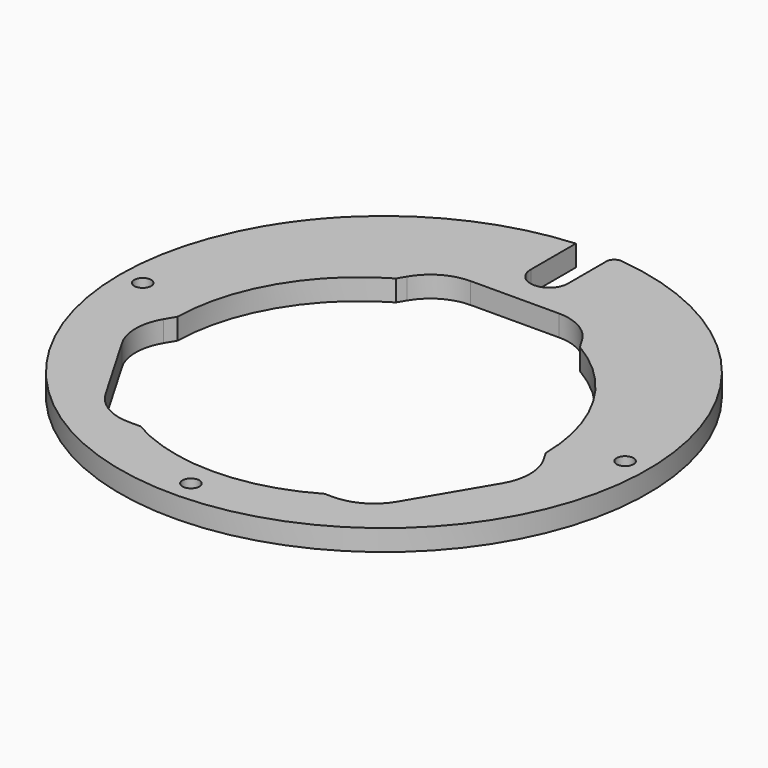
from build123d import *

# Parameters (mm, degrees)
F1_DEPTH = 4
F2_R     = 1.5
F3_R     = 1.6
F4_DEPTH = 4.001
F5_R     = 34.9
F6_DEPTH = 4.001


# Not quite as in the source:
# - a feature names something its author has since deleted; it is built from what else it names


with BuildPart() as f1:
    # F0 (on Top) → F1 (new body)
    with BuildSketch(Plane.XY):
        with BuildLine():
            ThreePointArc((-39.0789468534, 31.1903176135), (-41.1995846792, 28.3300939331), (-43.1112914302, 25.3262028584))
            ThreePointArc((-43.1112914302, 25.3262028584), (3.3909583102, -49.8848814947), (39.2874210825, 30.9273106604))
            ThreePointArc((39.2874210825, 30.9273106604), (23.4196994292, 44.1759853161), (3.5489706102, 49.8738890363))
            Line((3.5489706102, 49.8738890363), (3.5489706102, 39.2354845469))
            ThreePointArc((3.5489706102, 39.2354845469), (0, 35.6), (-3.5489706102, 39.2354845469))
            Line((-3.5489706102, 39.2354845469), (-3.5489706102, 49.8738890363))
            ThreePointArc((-3.5489706102, 49.8738890363), (-19.9954983208, 45.8277213802), (-34.1476646001, 36.5231023102))
            ThreePointArc((-34.1476646001, 36.5231023102), (-36.7102683781, 33.9463723482), (-39.0789468534, 31.1903176135))
        make_face()
        with BuildLine():
            Line((-36.0538297274, -7.1563580217), (-16.4297758662, 26.0448529843))
            ThreePointArc((-16.4297758662, 26.0448529843), (-12.9279784785, 29.4992312077), (-8.176710299, 30.7723237188))
            Line((-8.176710299, 30.7723237188), (8.4702026349, 30.8290335362))
            ThreePointArc((8.4702026349, 30.8290335362), (13.1364940427, 29.5958615472), (16.5612188168, 26.1949427186))
            Line((16.5612188168, 26.1949427186), (35.9620596652, -7.1371930753))
            ThreePointArc((35.9620596652, -7.1371930753), (37.2684771199, -12.0112511492), (35.9293854445, -16.8764337932))
            Line((35.9293854445, -16.8764337932), (27.4589141067, -31.2073110011))
            ThreePointArc((27.4589141067, -31.2073110011), (23.957116719, -34.6616892246), (19.2058485395, -35.9347817357))
            Line((19.2058485395, -35.9347817357), (-19.3610626759, -36.0661648035))
            ThreePointArc((-19.3610626759, -36.0661648035), (-24.1774760593, -34.793319721), (-27.7123796465, -31.2829879542))
            Line((-27.7123796465, -31.2829879542), (-36.0865039481, -16.8955987396))
            ThreePointArc((-36.0865039481, -16.8955987396), (-37.3929214028, -12.0215406656), (-36.0538297274, -7.1563580217))
        make_face(mode=Mode.SUBTRACT)
    extrude(amount=F1_DEPTH)

    # F2
    f2_edges = [f1.edges().sort_by_distance(p)[0] for p in [
        (39.287421, 30.927311, 2),
        (3.548971, 49.873889, 2),
    ]]
    fillet(f2_edges, radius=F2_R)

    # F3 (on face) → F4 (cut, through all)
    with BuildSketch(Plane.XY.offset(4)):
        with Locations((0, 45.69)):
            Circle(F3_R)
        with Locations((-45.69, 0)):
            Circle(F3_R)
        with Locations((0, -45.69)):
            Circle(F3_R)
        with Locations((45.69, 0)):
            Circle(F3_R)
    extrude(amount=-F4_DEPTH, mode=Mode.SUBTRACT)

    # F5 (on face) → F6 (cut, through all)
    with BuildSketch(Plane.XY.offset(4)):
        with Locations((0, -5.7566108276)):
            Circle(F5_R)
    extrude(amount=-F6_DEPTH, mode=Mode.SUBTRACT)


solid = f1.part
